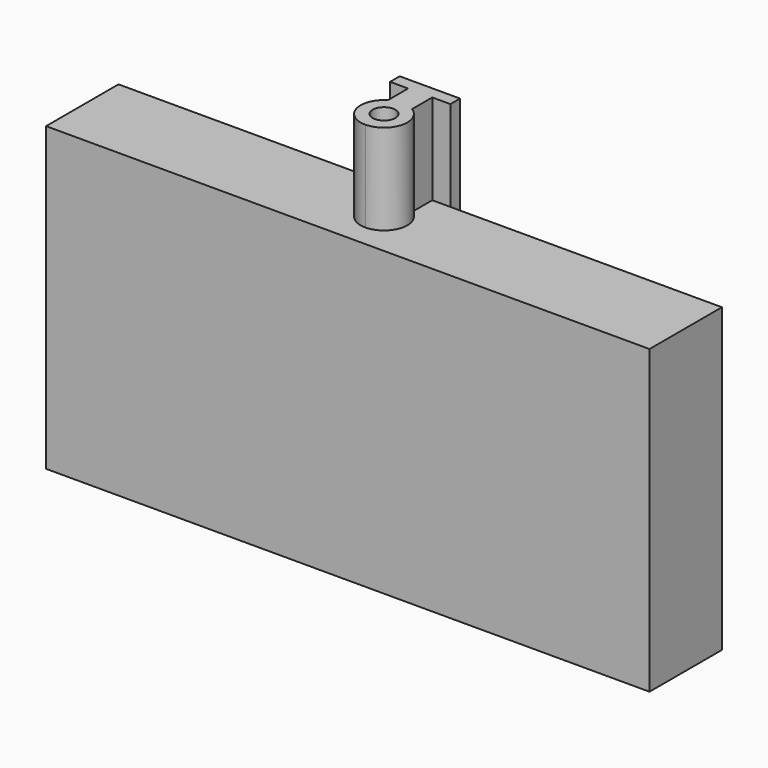
from build123d import *

# Parameters (mm, degrees)
F0_W     = 254
F0_H     = 38.1
F1_DEPTH = 127
F3_DEPTH = 38.1
F4_W     = 25.4
F4_H     = 5.08
F5_DEPTH = 38.1


with BuildPart() as f1:
    # F0 (on Top) → F1 (new body)
    with BuildSketch(Plane.XY):
        with Locations((0, -19.05)):
            Rectangle(F0_W, F0_H)
    extrude(amount=-F1_DEPTH)


with BuildPart() as f3:
    # F2 (on Top) → F3 (new body)
    with BuildSketch(Plane.XY):
        with BuildLine():
            ThreePointArc((-5.08, -10.6197920399), (-9.4828563233, -21.686331201), (0, -28.8925))
            ThreePointArc((0, -28.8925), (9.4828563233, -21.686331201), (5.08, -10.6197920399))
            Line((5.08, -10.6197920399), (5.08, 0))
            Line((5.08, 0), (12.7, 0))
            Line((12.7, 0), (12.7, 5.08))
            Line((12.7, 5.08), (-12.7, 5.08))
            Line((-12.7, 5.08), (-12.7, 0))
            Line((-12.7, 0), (-5.08, 0))
            Line((-5.08, 0), (-5.08, -10.6197920399))
        make_face()
        with BuildLine():
            ThreePointArc((0, -14.2875), (3.3675960454, -15.6824039546), (4.7625, -19.05))
            ThreePointArc((4.7625, -19.05), (3.3675960454, -22.4175960454), (0, -23.8125))
            ThreePointArc((0, -23.8125), (-4.7625, -19.05), (0, -14.2875))
        make_face(mode=Mode.SUBTRACT)
    extrude(amount=F3_DEPTH)

    # F4 (on face) → F5 (join)
    with BuildSketch(Plane(origin=(0, 0, 0), x_dir=(1, 0, 0), z_dir=(0, 0, -1))):
        with Locations((0, -2.54)):
            Rectangle(F4_W, F4_H)
    extrude(amount=F5_DEPTH)


solid = Compound([f1.part, f3.part])
